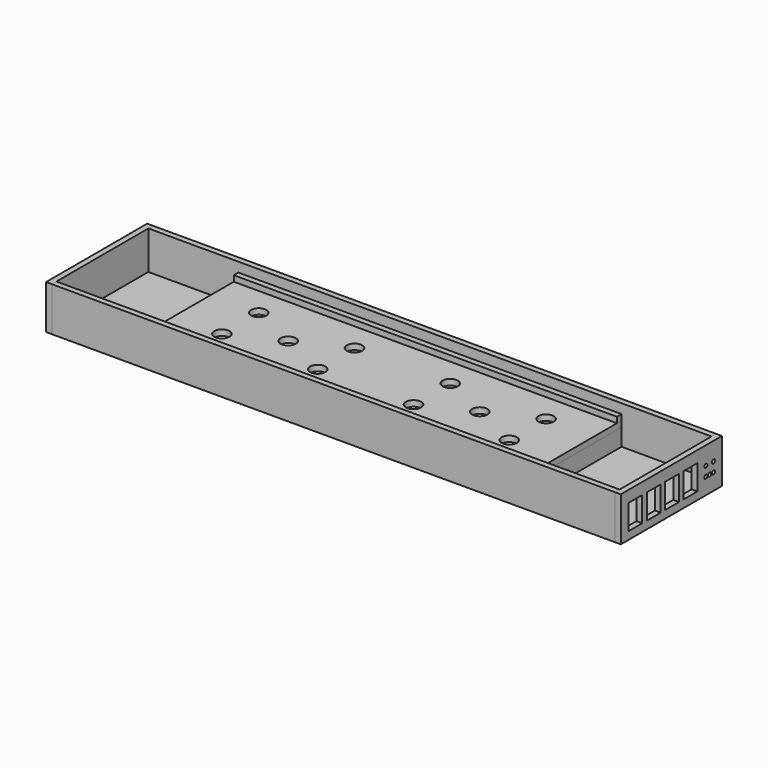
from build123d import *

# Parameters (mm, degrees)
F0_W      = 200
F0_H      = 60
F1_DEPTH  = 3
F2_W      = 3
F2_H      = 60
F3_DEPTH  = 9
F4_W      = 47
F4_H      = 60
F4_W_2    = 3
F5_DEPTH  = 3
F6_W      = 47
F6_H      = 60
F6_W_2    = 3
F7_DEPTH  = 3
F8_W      = 200
F8_H      = 3
F9_DEPTH  = 3
F10_R     = 4
F11_DEPTH = 3
F12_W     = 294
F12_H     = 23
F12_W_2   = 200
F12_H_2   = 3
F13_DEPTH = 3
F14_W     = 294
F14_H     = 23
F14_W_2   = 200
F14_H_2   = 3
F15_DEPTH = 3
F16_W     = 63
F16_H     = 23
F16_W_2   = 3
F17_DEPTH = 3
F18_W     = 3
F18_H     = 23
F18_W_2   = 63
F19_DEPTH = 3
F20_W     = 9
F20_H     = 13
F20_R     = 1
F21_DEPTH = 25


# Not quite as in the source:
# - a feature names something its author has since deleted; it is built from what else it names


with BuildPart() as f1:
    # F0 (on Top) → F1 (new body)
    with BuildSketch(Plane.XY):
        Rectangle(F0_W, F0_H)
    extrude(amount=F1_DEPTH)

    # F10 (on face) → F11 (cut)
    with BuildSketch(Plane.XY.offset(3)):
        with Locations((-75, 12)):
            Circle(F10_R)
        with Locations((-75, -12)):
            Circle(F10_R)
        with Locations((-25, -12)):
            Circle(F10_R)
        with Locations((-25, 12)):
            Circle(F10_R)
        with Locations((25, 12)):
            Circle(F10_R)
        with Locations((25, -12)):
            Circle(F10_R)
        with Locations((50, 0)):
            Circle(F10_R)
        with Locations((75, 12)):
            Circle(F10_R)
        with Locations((75, -12)):
            Circle(F10_R)
        with Locations((-50, 0)):
            Circle(F10_R)
    extrude(amount=-F11_DEPTH, mode=Mode.SUBTRACT)


with BuildPart() as f3:
    # F2 (on face) → F3 (new body)
    with BuildSketch(Plane(origin=(0, 0, 0), x_dir=(1, 0, 0), z_dir=(0, 0, -1))):
        with Locations((-98.5, 0)):
            Rectangle(F2_W, F2_H)
    extrude(amount=F3_DEPTH)


with BuildPart() as f3b:
    # F2 (on face) → F3, piece 2 (new body)
    with BuildSketch(Plane(origin=(0, 0, 0), x_dir=(1, 0, 0), z_dir=(0, 0, -1))):
        with Locations((98.5, 0)):
            Rectangle(F2_W, F2_H)
    extrude(amount=F3_DEPTH)


with BuildPart() as f5:
    # F4 (on face) → F5 (new body)
    with BuildSketch(Plane(origin=(0, 0, -9), x_dir=(1, 0, 0), z_dir=(0, 0, -1))):
        with Locations((123.5, 0)):
            Rectangle(F4_W, F4_H)
        with Locations((98.5, 0)):
            Rectangle(F4_W_2, F4_H)
    extrude(amount=F5_DEPTH)


with BuildPart() as f7:
    # F6 (on face) → F7 (new body)
    with BuildSketch(Plane(origin=(0, 0, -9), x_dir=(1, 0, 0), z_dir=(0, 0, -1))):
        with Locations((-123.5, 0)):
            Rectangle(F6_W, F6_H)
        with Locations((-98.5, 0)):
            Rectangle(F6_W_2, F6_H)
    extrude(amount=F7_DEPTH)


with BuildPart() as f9:
    # F8 (on face) → F9 (new body)
    with BuildSketch(Plane.XY.offset(3)):
        with Locations((0, 28.5)):
            Rectangle(F8_W, F8_H)
    extrude(amount=F9_DEPTH)


with BuildPart() as f9b:
    # F8 (on face) → F9, piece 2 (new body)
    with BuildSketch(Plane.XY.offset(3)):
        with Locations((0, -28.5)):
            Rectangle(F8_W, F8_H)
    extrude(amount=F9_DEPTH)


with BuildPart() as f13:
    # F12 (on face) → F13 (new body)
    with BuildSketch(Plane.XZ.offset(30)):
        with Locations((0, -0.5)):
            Rectangle(F12_W, F12_H)
        with Locations((0, 1.5)):
            Rectangle(F12_W_2, F12_H_2, mode=Mode.SUBTRACT)
        with Locations((0, 1.5)):
            Rectangle(F12_W_2, F12_H_2)
    extrude(amount=F13_DEPTH)


with BuildPart() as f15:
    # F14 (on face) → F15 (new body)
    with BuildSketch(Plane(origin=(0, 30, 0), x_dir=(-1, 0, 0), z_dir=(0, 1, 0))):
        with Locations((0, -0.5)):
            Rectangle(F14_W, F14_H)
        with Locations((0, 1.5)):
            Rectangle(F14_W_2, F14_H_2, mode=Mode.SUBTRACT)
        with Locations((0, 1.5)):
            Rectangle(F14_W_2, F14_H_2)
    extrude(amount=F15_DEPTH)


with BuildPart() as f17:
    # F16 (on face) → F17 (new body)
    with BuildSketch(Plane.YZ.offset(147)):
        with Locations((1.5, -0.5)):
            Rectangle(F16_W, F16_H)
        with Locations((-31.5, -0.5)):
            Rectangle(F16_W_2, F16_H)
    extrude(amount=F17_DEPTH)

    # F20 (on face) → F21 (cut)
    with BuildSketch(Plane.YZ.offset(150)):
        with Locations((-23.5, -1.5)):
            Rectangle(F20_W, F20_H)
        with Locations((-11.5, -1.5)):
            Rectangle(F20_W, F20_H)
        with Locations((0.5, -1.5)):
            Rectangle(F20_W, F20_H)
        with Locations((12.5, -1.5)):
            Rectangle(F20_W, F20_H)
        with Locations((22.5, 1.5)):
            Circle(F20_R)
        with Locations((27.5, 1.5)):
            Circle(F20_R)
        with Locations((27.5, -3.5)):
            Circle(F20_R)
        with Locations((25, -3.5)):
            Circle(F20_R)
        with Locations((22.5, -3.5)):
            Circle(F20_R)
    extrude(amount=-F21_DEPTH, mode=Mode.SUBTRACT)


with BuildPart() as f19:
    # F18 (on face) → F19 (new body)
    with BuildSketch(Plane(origin=(-147, 0, 0), x_dir=(0, -1, 0), z_dir=(-1, 0, 0))):
        with Locations((-31.5, -0.5)):
            Rectangle(F18_W, F18_H)
        with Locations((1.5, -0.5)):
            Rectangle(F18_W_2, F18_H)
    extrude(amount=F19_DEPTH)


solid = Compound([f1.part, f3.part, f3b.part, f5.part, f7.part, f9.part, f9b.part, f13.part, f15.part, f17.part, f19.part])
